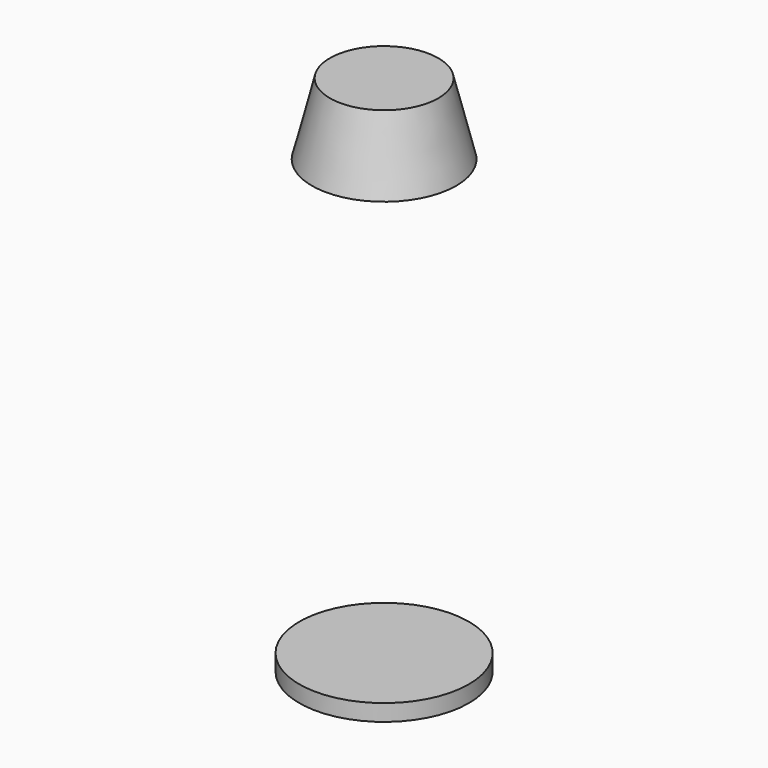
from build123d import *

# Parameters (mm, degrees)
F0_R     = 7.055
F1_DEPTH = 1.38
F7_R     = 4.515
F4_R     = 6.005


# Not quite as in the source:
# - the program builds the solid bodies; features that only make, move or delete a surface that nothing else refers to are left out


with BuildPart() as f1:
    # F0 (on Top) → F1 (new body)
    with BuildSketch(Plane.XY):
        Circle(F0_R)
    extrude(amount=F1_DEPTH)


with BuildPart() as f9:
    # F7 (on offset) → F9 section 0
    with BuildSketch(Plane.XY.offset(43.4796)):
        Circle(F7_R)
    # F4 (on offset) → F9 section 1
    with BuildSketch(Plane.XY.offset(37.5496)):
        Circle(F4_R)
    loft()


solid = Compound([f1.part, f9.part])
